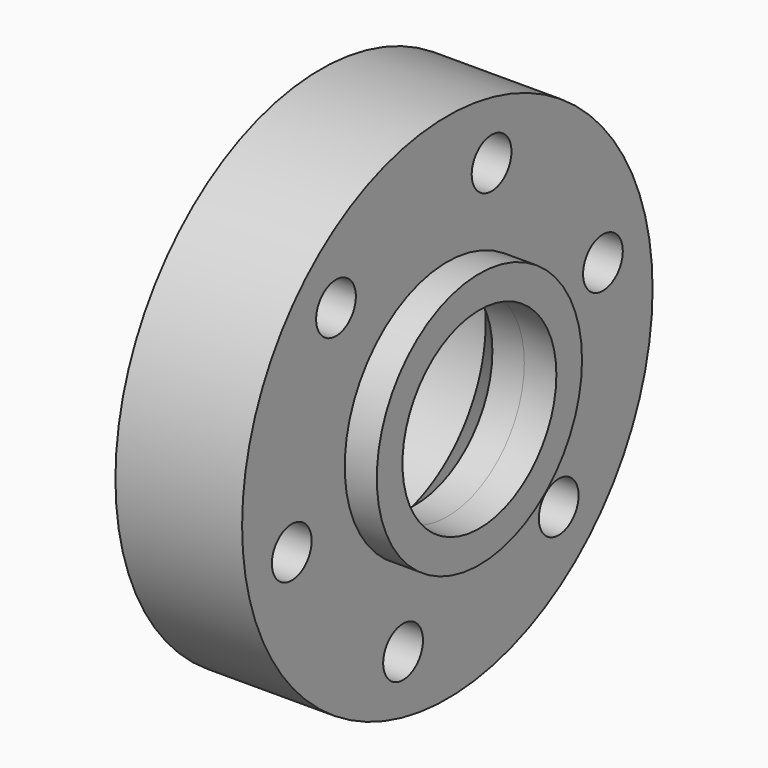
from build123d import *

# Parameters (mm, degrees)
F0_R            = 16
F1_DEPTH        = 7.9
F2_R            = 8.11
F3_DEPTH        = 3.8
F4_R            = 6
F5_DEPTH        = 7.901
F6_R            = 1.55
F7_DEPTH        = 7.901
F7_COPIES_COUNT = 6
F8_R            = 8
F8_R_2          = 6
F9_DEPTH        = 2
F10_SIZE2       = 2.10999
F10_SIZE        = 2.10999


# Not quite as in the source:
# - a fillet or chamfer is up to 0.001 mm smaller than in the source, because OpenCascade refuses the exact size
# - a pattern or mirror of a feature is missing from the dataset's text; its kind, count and spacing are read off the source's solid


with BuildPart() as f1:
    # F0 (on Right) → F1 (new body)
    with BuildSketch(Plane.YZ):
        Circle(F0_R)
    extrude(amount=F1_DEPTH)

    # F2 (on face) → F3 (cut)
    with BuildSketch(Plane(origin=(0, 0, 0), x_dir=(0, -1, 0), z_dir=(-1, 0, 0))):
        Circle(F2_R)
    extrude(amount=-F3_DEPTH, mode=Mode.SUBTRACT)

    # F4 (on face) → F5 (cut, through all)
    with BuildSketch(Plane.YZ.offset(7.9)):
        Circle(F4_R)
    extrude(amount=-F5_DEPTH, mode=Mode.SUBTRACT)

    # F6 (on face) → F7 (cut, through all)
    with BuildSketch(Plane(origin=(0, 0, 0), x_dir=(0, -1, 0), z_dir=(-1, 0, 0))):
        with Locations((-3.4491492906, 12.0147146937)):
            Circle(F6_R)
    f7 = extrude(amount=-F7_DEPTH, mode=Mode.SUBTRACT)

    # F7_copies: F7 ×6 about axis
    f7_copies_axis = Axis((0, 0, 0), (1, 0, 0))
    for i in range(1, F7_COPIES_COUNT):
        add(f7.rotate(f7_copies_axis, i * 360 / F7_COPIES_COUNT), mode=Mode.SUBTRACT)

    # F8 (on face) → F9 (join)
    with BuildSketch(Plane.YZ.offset(7.9)):
        Circle(F8_R)
        Circle(F8_R_2, mode=Mode.SUBTRACT)
    extrude(amount=F9_DEPTH)

    # F10 (size 2.11 and 2.11 in the source; OpenCascade refuses exactly that, so slightly less here)
    f10_edges = [f1.edges().sort_by_distance(p)[0] for p in [
        (3.8, -6, 0),
    ]]
    chamfer(f10_edges, length=F10_SIZE, length2=F10_SIZE2)


solid = f1.part
